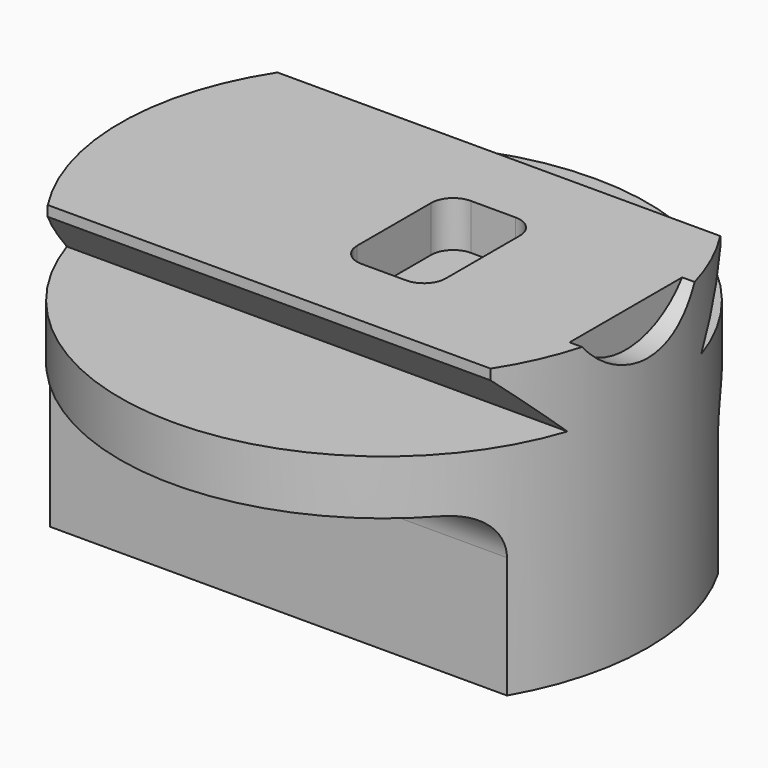
from build123d import *

# Parameters (mm, degrees)
F0_R      = 19.05
F1_DEPTH  = 20.955
F3_DEPTH  = 25.4
F5_DEPTH  = 25.4
F6_R      = 4.572
F7_DEPTH  = 17.145
F9_D      = 3.4544
F9_DEPTH  = 10.81405
F9_TIP    = 1.0378064612
F11_R     = 6.35
F12_DEPTH = 1.5875
F14_DEPTH = 3.302


# Not quite as in the source:
# - a feature names something its author has since deleted; it is built from what else it names


with BuildPart() as f1:
    # F0 (on Top) → F1 (new body)
    with BuildSketch(Plane.XY):
        Circle(F0_R)
    extrude(amount=-F1_DEPTH)

    # F2 (on Right) → F3 (cut, symmetric)
    with BuildSketch(Plane.YZ):
        Polygon((-10.3632, -0.7493), (-10.3632, 0), (-19.05, 0), (-19.05, -5.08), (-6.0325, -5.08), align=None)
        Polygon((10.3632, -0.7493), (6.0325, -5.08), (19.05, -5.08), (19.05, 0), (10.3632, 0), align=None)
    extrude(amount=F3_DEPTH, both=True, mode=Mode.SUBTRACT)

    # F4 (on Right) → F5 (cut, symmetric)
    with BuildSketch(Plane.YZ):
        with BuildLine():
            Line((-19.05, -20.955), (-9.525, -20.955))
            Line((-9.525, -20.955), (-9.525, -12.192))
            ThreePointArc((-9.525, -12.192), (-10.4549359697, -9.9469359697), (-12.7, -9.017))
            Line((-12.7, -9.017), (-19.05, -9.017))
            Line((-19.05, -9.017), (-19.05, -20.955))
        make_face()
        with BuildLine():
            Line((19.05, -9.017), (12.7, -9.017))
            ThreePointArc((12.7, -9.017), (10.4549359697, -9.9469359697), (9.525, -12.192))
            Line((9.525, -12.192), (9.525, -20.955))
            Line((9.525, -20.955), (19.05, -20.955))
            Line((19.05, -20.955), (19.05, -9.017))
        make_face()
    extrude(amount=F5_DEPTH, both=True, mode=Mode.SUBTRACT)

    # F6 (on face) → F7 (cut)
    with BuildSketch(Plane(origin=(0, 0, -20.955), x_dir=(1, 0, 0), z_dir=(0, 0, -1))):
        Circle(F6_R)
        with Locations((-11.684, 0)):
            Circle(F6_R)
    extrude(amount=-F7_DEPTH, mode=Mode.SUBTRACT)

    # F9
    with Locations(Plane(origin=(0, 9.525, 0), x_dir=(-1, 0, 0), z_dir=(0, 1, 0))):
        with Locations((0, -14.2748), (11.684, -14.2748)):
            Hole(F9_D / 2, depth=F9_DEPTH)
            with Locations((0, 0, -(F9_DEPTH + F9_TIP / 2))):  # 118° drill point
                Cone(0, F9_D / 2, F9_TIP, mode=Mode.SUBTRACT)

    # F11 (on offset) → F12 (cut)
    with BuildSketch(Plane.YZ.offset(19.05)):
        with Locations((0, 3.81)):
            Circle(F11_R)
    extrude(amount=-F12_DEPTH, mode=Mode.SUBTRACT)

    # F13 (on face) → F14 (cut)
    with BuildSketch(Plane.XY):
        with BuildLine():
            Line((5.5499, 4.9276), (2.3241, 4.9276))
            ThreePointArc((2.3241, 4.9276), (1.2015679849, 4.4626320151), (0.7366, 3.3401))
            Line((0.7366, 3.3401), (0.7366, -3.3401))
            ThreePointArc((0.7366, -3.3401), (1.2015679849, -4.4626320151), (2.3241, -4.9276))
            Line((2.3241, -4.9276), (5.5499, -4.9276))
            ThreePointArc((5.5499, -4.9276), (6.6724320151, -4.4626320151), (7.1374, -3.3401))
            Line((7.1374, -3.3401), (7.1374, 3.3401))
            ThreePointArc((7.1374, 3.3401), (6.6724320151, 4.4626320151), (5.5499, 4.9276))
        make_face()
    extrude(amount=-F14_DEPTH, mode=Mode.SUBTRACT)


solid = f1.part
